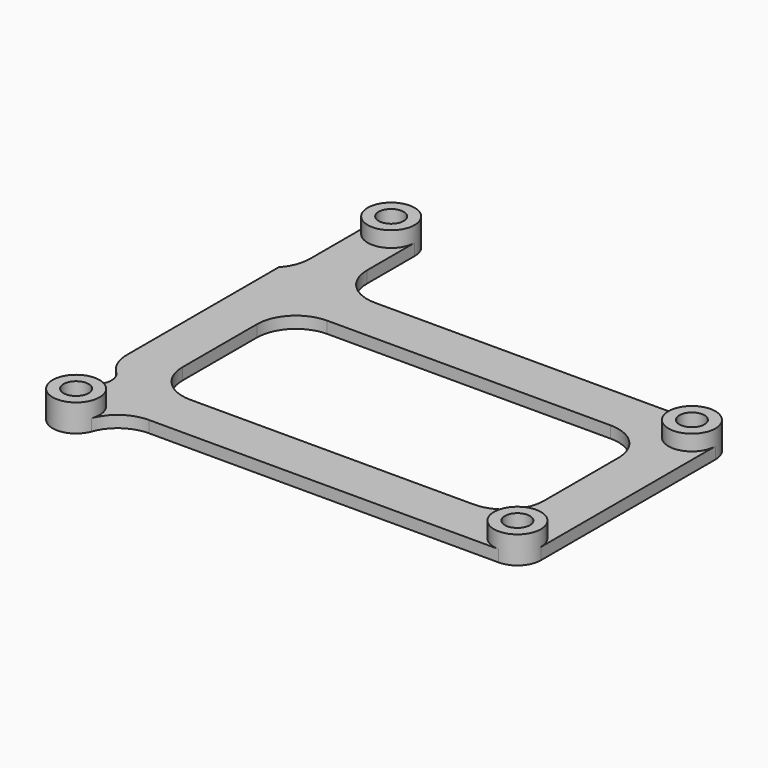
from build123d import *

# Parameters (mm, degrees)
F0_R        = 1.6
F1_DEPTH    = 1.5
F2_DEPTH    = 3.5
F3_T1_DEPTH = 1.5
F4_R        = 5


# Not quite as in the source:
# - a fillet or chamfer that OpenCascade refuses, or shapes differently, is made with other operations: its cross-section is extruded or revolved along the edge and cut away or added
# - a feature names something its author has since deleted; it is built from what else it names


with BuildPart() as f1:
    # F0 (on Top) → F1 (new body)
    with BuildSketch(Plane.XY):
        with BuildLine():
            Line((-18.9040250808, 5.7581766099), (-18.9040250808, 11.7581766099))
            Line((-18.9040250808, 11.7581766099), (-23.6040250808, 11.7581766099))
            Line((-23.6040250808, 11.7581766099), (-24.9040250808, 11.7581766099))
            Line((-24.9040250808, 11.7581766099), (-24.9040250808, -15.541421883))
            ThreePointArc((-24.9040250808, -15.541421883), (-22.6536235737, -17.7918233901), (-24.9040250808, -20.0422248973))
            Line((-24.9040250808, -20.0422248973), (-24.9040250808, -24.3918233901))
            ThreePointArc((-24.9040250808, -24.3918233901), (-21.9040250808, -21.3918233901), (-18.9040250808, -24.3918233901))
            Line((-18.9040250808, -24.3918233901), (-18.9040250808, -22.1418233901))
            Line((-18.9040250808, -22.1418233901), (-18.9040250808, -16.1418233901))
            Line((-18.9040250808, -16.1418233901), (-18.9040250808, 5.7581766099))
        make_face()
        with BuildLine():
            ThreePointArc((33.3459749192, 8.7581766099), (28.2246545756, 6.6368562663), (30.3459749192, 11.7581766099))
            Line((30.3459749192, 11.7581766099), (-17.6040250808, 11.7581766099))
            Line((-17.6040250808, 11.7581766099), (-18.9040250808, 11.7581766099))
            Line((-18.9040250808, 11.7581766099), (-18.9040250808, 5.7581766099))
            Line((-18.9040250808, 5.7581766099), (27.3459749192, 5.7581766099))
            Line((27.3459749192, 5.7581766099), (27.3459749192, -16.1418233901))
            Line((27.3459749192, -16.1418233901), (-18.9040250808, -16.1418233901))
            Line((-18.9040250808, -16.1418233901), (-18.9040250808, -22.1418233901))
            Line((-18.9040250808, -22.1418233901), (30.3459749192, -22.1418233901))
            ThreePointArc((30.3459749192, -22.1418233901), (28.2246545756, -17.0205030466), (33.3459749192, -19.1418233901))
            Line((33.3459749192, -19.1418233901), (33.3459749192, 8.7581766099))
        make_face()
        with BuildLine():
            ThreePointArc((-24.9040250808, -24.3918233901), (-21.9040250808, -27.3918233901), (-18.9040250808, -24.3918233901))
            ThreePointArc((-18.9040250808, -24.3918233901), (-21.9040250808, -21.3918233901), (-24.9040250808, -24.3918233901))
        make_face()
        with Locations((-21.9040250808, -24.3918233901)):
            Circle(F0_R, mode=Mode.SUBTRACT)
        with BuildLine():
            ThreePointArc((30.3459749192, -22.1418233901), (32.4672952628, -21.2631437337), (33.3459749192, -19.1418233901))
            ThreePointArc((33.3459749192, -19.1418233901), (28.2246545756, -17.0205030466), (30.3459749192, -22.1418233901))
        make_face()
        with Locations((30.3459749192, -19.1418233901)):
            Circle(F0_R, mode=Mode.SUBTRACT)
        with BuildLine():
            ThreePointArc((33.3459749192, 8.7581766099), (32.4672952628, 10.8794969534), (30.3459749192, 11.7581766099))
            ThreePointArc((30.3459749192, 11.7581766099), (28.2246545756, 6.6368562663), (33.3459749192, 8.7581766099))
        make_face()
        with Locations((30.3459749192, 8.7581766099)):
            Circle(F0_R, mode=Mode.SUBTRACT)
        with BuildLine():
            Line((-18.9040250808, 11.7581766099), (-17.6040250808, 11.7581766099))
            Line((-17.6040250808, 11.7581766099), (-17.6040250808, 24.3581766099))
            ThreePointArc((-17.6040250808, 24.3581766099), (-20.6040250808, 21.3581766099), (-23.6040250808, 24.3581766099))
            Line((-23.6040250808, 24.3581766099), (-23.6040250808, 11.7581766099))
            Line((-23.6040250808, 11.7581766099), (-18.9040250808, 11.7581766099))
        make_face()
        with BuildLine():
            ThreePointArc((-23.6040250808, 24.3581766099), (-20.6040250808, 21.3581766099), (-17.6040250808, 24.3581766099))
            ThreePointArc((-17.6040250808, 24.3581766099), (-20.6040250808, 27.3581766099), (-23.6040250808, 24.3581766099))
        make_face()
        with Locations((-20.6040250808, 24.3581766099)):
            Circle(F0_R, mode=Mode.SUBTRACT)
    extrude(amount=F1_DEPTH)

    # F0 (on Top) → F2 (join)
    with BuildSketch(Plane.XY):
        with BuildLine():
            ThreePointArc((-24.9040250808, -24.3918233901), (-21.9040250808, -27.3918233901), (-18.9040250808, -24.3918233901))
            ThreePointArc((-18.9040250808, -24.3918233901), (-21.9040250808, -21.3918233901), (-24.9040250808, -24.3918233901))
        make_face()
        with Locations((-21.9040250808, -24.3918233901)):
            Circle(F0_R, mode=Mode.SUBTRACT)
        with BuildLine():
            ThreePointArc((33.3459749192, 8.7581766099), (32.4672952628, 10.8794969534), (30.3459749192, 11.7581766099))
            ThreePointArc((30.3459749192, 11.7581766099), (28.2246545756, 6.6368562663), (33.3459749192, 8.7581766099))
        make_face()
        with Locations((30.3459749192, 8.7581766099)):
            Circle(F0_R, mode=Mode.SUBTRACT)
        with BuildLine():
            ThreePointArc((30.3459749192, -22.1418233901), (32.4672952628, -21.2631437337), (33.3459749192, -19.1418233901))
            ThreePointArc((33.3459749192, -19.1418233901), (28.2246545756, -17.0205030466), (30.3459749192, -22.1418233901))
        make_face()
        with Locations((30.3459749192, -19.1418233901)):
            Circle(F0_R, mode=Mode.SUBTRACT)
        with BuildLine():
            ThreePointArc((-23.6040250808, 24.3581766099), (-20.6040250808, 21.3581766099), (-17.6040250808, 24.3581766099))
            ThreePointArc((-17.6040250808, 24.3581766099), (-20.6040250808, 27.3581766099), (-23.6040250808, 24.3581766099))
        make_face()
        with Locations((-20.6040250808, 24.3581766099)):
            Circle(F0_R, mode=Mode.SUBTRACT)
    extrude(amount=F2_DEPTH)

    # F3: fillet of radius 5 on 7 edges, made by hand

    # F3_s2 → F3_t1 (join)
    with BuildSketch(Plane.XY):
        with BuildLine():
            ThreePointArc((-18.9040250808, 0.7581766099), (-17.4395589867, 4.2937105158), (-13.9040250808, 5.7581766099))
            Line((-13.9040250808, 5.7581766099), (-18.9040250808, 5.7581766099))
            Line((-18.9040250808, 5.7581766099), (-18.9040250808, 0.7581766099))
        make_face()
        with BuildLine():
            ThreePointArc((-18.9040250808, -11.1418233901), (-17.4395589867, -14.6773572961), (-13.9040250808, -16.1418233901))
            Line((-13.9040250808, -16.1418233901), (-18.9040250808, -16.1418233901))
            Line((-18.9040250808, -16.1418233901), (-18.9040250808, -11.1418233901))
        make_face()
        with BuildLine():
            ThreePointArc((22.3459749192, 5.7581766099), (25.8815088251, 4.2937105158), (27.3459749192, 0.7581766099))
            Line((27.3459749192, 0.7581766099), (27.3459749192, 5.7581766099))
            Line((27.3459749192, 5.7581766099), (22.3459749192, 5.7581766099))
        make_face()
        with BuildLine():
            ThreePointArc((22.3459749192, -16.1418233901), (25.8815088251, -14.6773572961), (27.3459749192, -11.1418233901))
            Line((27.3459749192, -11.1418233901), (27.3459749192, -16.1418233901))
            Line((27.3459749192, -16.1418233901), (22.3459749192, -16.1418233901))
        make_face()
        with BuildLine():
            ThreePointArc((-17.6040250808, 16.7581766099), (-16.1395589867, 13.2226427039), (-12.6040250808, 11.7581766099))
            Line((-12.6040250808, 11.7581766099), (-17.6040250808, 11.7581766099))
            Line((-17.6040250808, 11.7581766099), (-17.6040250808, 16.7581766099))
        make_face()
        with BuildLine():
            ThreePointArc((-24.9040250808, 11.7581766099), (-23.9403355543, 13.3184353163), (-23.6040250808, 15.121210954))
            Line((-23.6040250808, 15.121210954), (-23.6040250808, 11.7581766099))
            Line((-23.6040250808, 11.7581766099), (-24.9040250808, 11.7581766099))
        make_face()
        with BuildLine():
            ThreePointArc((-19.0868414806, -25.4230733901), (-17.2556452895, -23.0434243124), (-14.3915354801, -22.1418233901))
            Line((-14.3915354801, -22.1418233901), (-14.3915354801, -21.6418233901))
            Line((-14.3915354801, -21.6418233901), (-18.9040250808, -21.6418233901))
            Line((-18.9040250808, -21.6418233901), (-19.4040250808, -22.1418233901))
            ThreePointArc((-19.4040250808, -22.1418233901), (-19.4040250808, -24.3918233901), (-19.5563720806, -25.2511983901))
            Line((-19.5563720806, -25.2511983901), (-19.0868414806, -25.4230733901))
        make_face()
    extrude(amount=F3_T1_DEPTH)

    # F4
    f4_edges = [f1.edges().sort_by_distance(p)[0] for p in [
        (-24.904025, -15.541422, 0.75),
        (-24.904025, -20.042225, 0.75),
    ]]
    fillet(f4_edges, radius=F4_R)


solid = f1.part
